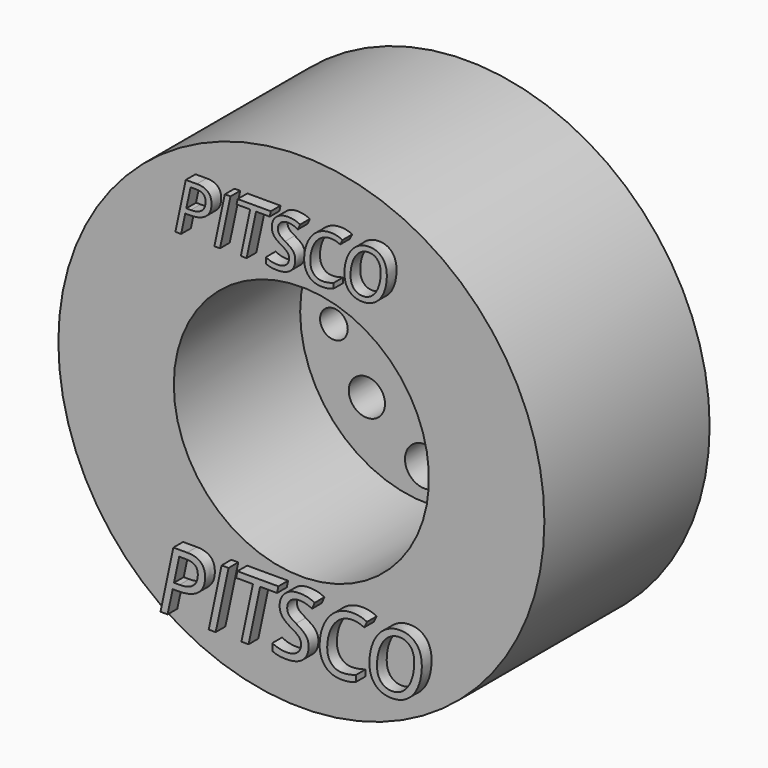
from build123d import *

# Parameters (mm, degrees)
F1_DEPTH     = 17
F3_DEPTH     = 13
F5_DEPTH     = 14
F6_R         = 1.3923187955
F6_R_2       = 1.2883465455
F6_R_3       = 1.6132517616
F6_R_4       = 1.1391885134
F6_R_5       = 1.4913239272
F6_R_6       = 1.4998455073
F6_R_7       = 1.5965746889
F6_R_8       = 1.487901156
F7_DEPTH     = 25
F9_TEXT_SIZE = 7.0017477911
F8_TEXT_SIZE = 5.6650179128
F10_DEPTH    = 1
F11_R        = 2.0949058831
F12_DEPTH    = 13
F13_R        = 2.0420394001
F14_DEPTH    = 13


# Not quite as in the source:
# - Text() gives the source's letters only with a copy of the font that has no kerning and outlines rounded to 1/6400 em; it was checked with that copy


with BuildPart() as f1:
    # F0 (on Front) → F1 (new body)
    with BuildSketch(Plane.XZ):
        with BuildLine():
            ThreePointArc((6.7942569819, 0), (26.7942569819, -20), (46.7942569819, 0))
            Line((46.7942569819, 0), (6.7942569819, 0))
        make_face()
        with BuildLine():
            Line((6.7942569819, 0), (46.7942569819, 0))
            ThreePointArc((46.7942569819, 0), (26.7942569819, 20), (6.7942569819, 0))
        make_face()
    extrude(amount=F1_DEPTH)

    # F2 (on face) → F3 (cut)
    with BuildSketch(Plane.XZ.offset(17)):
        with BuildLine():
            Line((16.2942569819, 0), (37.2942569819, 0))
            ThreePointArc((37.2942569819, 0), (26.7942569819, 10.5), (16.2942569819, 0))
        make_face()
        with BuildLine():
            ThreePointArc((16.2942569819, 0), (26.7942569819, -10.5), (37.2942569819, 0))
            Line((37.2942569819, 0), (16.2942569819, 0))
        make_face()
    extrude(amount=-F3_DEPTH, mode=Mode.SUBTRACT)

    # F4 (on face) → F5 (join)
    with BuildSketch(Plane(origin=(0, 0, 0), x_dir=(-1, 0, 0), z_dir=(0, 1, 0))):
        with BuildLine():
            Line((-29.7942569819, 0), (-23.7942569819, 0))
            ThreePointArc((-23.7942569819, 0), (-26.7942569819, 3), (-29.7942569819, 0))
        make_face()
        with BuildLine():
            ThreePointArc((-29.7942569819, 0), (-26.7942569819, -3), (-23.7942569819, 0))
            Line((-23.7942569819, 0), (-29.7942569819, 0))
        make_face()
    extrude(amount=F5_DEPTH)

    # F6 (on face) → F7 (cut)
    with BuildSketch(Plane.XZ.offset(4)):
        with Locations((26.5338011086, 8.0442298204)):
            Circle(F6_R)
        with Locations((33.9952036738, 0)):
            Circle(F6_R_2)
        with Locations((26.5338011086, -7.8781843185)):
            Circle(F6_R_3)
        with Locations((19.0724022686, 0)):
            Circle(F6_R_4)
        with Locations((21.7856373638, -4.4152378105)):
            Circle(F6_R_5)
        with Locations((32.5314812362, -4.8079430126)):
            Circle(F6_R_6)
        with Locations((31.4961671829, 5.580897443)):
            Circle(F6_R_7)
        with Locations((21.6428358108, 5.1881917752)):
            Circle(F6_R_8)
    extrude(amount=-F7_DEPTH, mode=Mode.SUBTRACT)

    # F9 (on face) + F8 (on face) → F10 (join)
    with BuildSketch(Plane.XZ.offset(17)):
        with Locations((15.7091179863, -16.1513071507)):
            Text('PITSCO', F9_TEXT_SIZE, font='Open Sans', font_style=FontStyle.ITALIC, text_align=(TextAlign.LEFT, TextAlign.BOTTOM))
    with BuildSketch(Plane.XZ.offset(17)):
        with Locations((16.990499571, 11.7738191038)):
            Text('PITSCO', F8_TEXT_SIZE, font='Open Sans', font_style=FontStyle.ITALIC, text_align=(TextAlign.LEFT, TextAlign.BOTTOM))
    extrude(amount=F10_DEPTH)

    # F11 (on face) → F12 (cut)
    with BuildSketch(Plane(origin=(0, 14, 0), x_dir=(-1, 0, 0), z_dir=(0, 1, 0))):
        with Locations((-26.7942569819, 0)):
            Circle(F11_R)
    extrude(amount=F12_DEPTH, mode=Mode.SUBTRACT)

    # F13 (on face) → F14 (cut)
    with BuildSketch(Plane(origin=(0, 14, 0), x_dir=(-1, 0, 0), z_dir=(0, 1, 0))):
        with Locations((-26.7942569819, 0)):
            Circle(F13_R)
    extrude(amount=-F14_DEPTH, mode=Mode.SUBTRACT)


solid = f1.part
